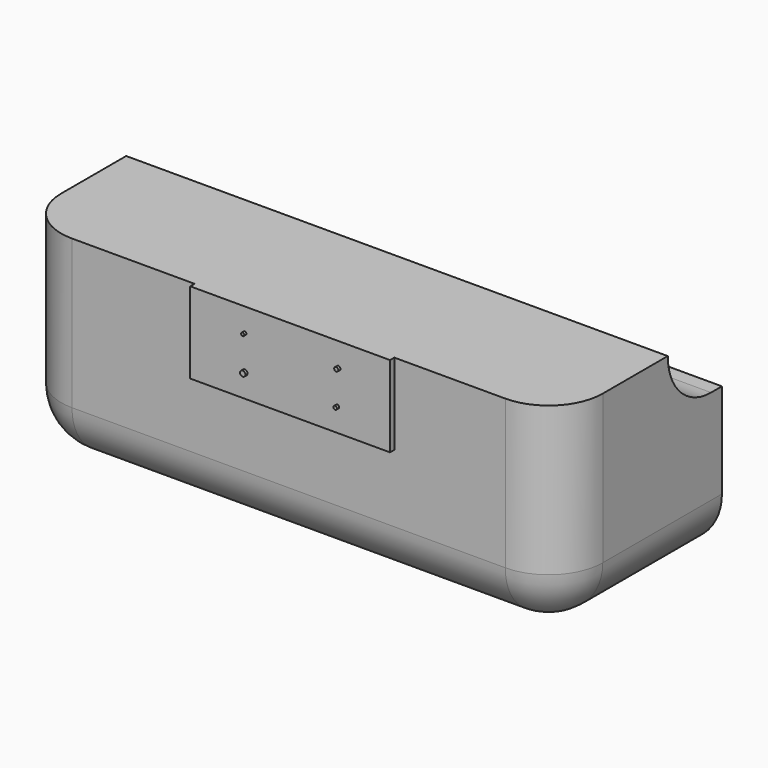
from build123d import *

# Parameters (mm, degrees)
F0_W     = 50.8
F0_H     = 19.05
F1_DEPTH = 19.05
F2_R     = 5.08
F3_R     = 5.08
F4_W     = 18.7399210408
F4_H     = 7.62
F5_DEPTH = 0.508
F6_R     = 0.1690866305
F6_R_2   = 0.254
F6_R_3   = 0.1908338751
F6_R_4   = 0.1508847562
F7_DEPTH = 0.254
F8_W     = 6.35
F8_H     = 5.08
F9_DEPTH = 50.8
F10_R    = 5.07999


# Not quite as in the source:
# - a fillet or chamfer is up to 0.001 mm smaller than in the source, because OpenCascade refuses the exact size


with BuildPart() as f1:
    # F0 (on Top) → F1 (new body)
    with BuildSketch(Plane.XY):
        Rectangle(F0_W, F0_H)
    extrude(amount=F1_DEPTH)

    # F2
    f2_edges = [f1.edges().sort_by_distance(p)[0] for p in [
        (-25.4, -9.525, 9.525),
        (25.4, -9.525, 9.525),
    ]]
    fillet(f2_edges, radius=F2_R)

    # F3
    f3_edges = [f1.edges().sort_by_distance(p)[0] for p in [
        (25.4, 2.54, 0),
    ]]
    fillet(f3_edges, radius=F3_R)

    # F4 (on face) → F5 (join)
    with BuildSketch(Plane.XZ.offset(9.525)):
        with Locations((0.5450607277, 15.24)):
            Rectangle(F4_W, F4_H)
    extrude(amount=F5_DEPTH)

    # F6 (on face) → F7 (join)
    with BuildSketch(Plane.XZ.offset(10.033)):
        with Locations((4.971065205, 13.6094420754)):
            Circle(F6_R)
        with Locations((-3.7048892478, 13.6058607324)):
            Circle(F6_R_2)
        with Locations((5.0740026747, 16.8156122121)):
            Circle(F6_R_3)
        with Locations((-3.7048892478, 16.8490853095)):
            Circle(F6_R_4)
    extrude(amount=F7_DEPTH)

    # F8 (on face) → F9 (cut)
    with BuildSketch(Plane.YZ.offset(25.4)):
        with Locations((6.35, 16.51)):
            Rectangle(F8_W, F8_H)
    extrude(amount=-F9_DEPTH, mode=Mode.SUBTRACT)

    # F10 (radius 5.08 in the source; OpenCascade refuses exactly that, so slightly less here)
    f10_edges = [f1.edges().sort_by_distance(p)[0] for p in [
        (0, 3.175, 13.97),
    ]]
    fillet(f10_edges, radius=F10_R)


solid = f1.part
